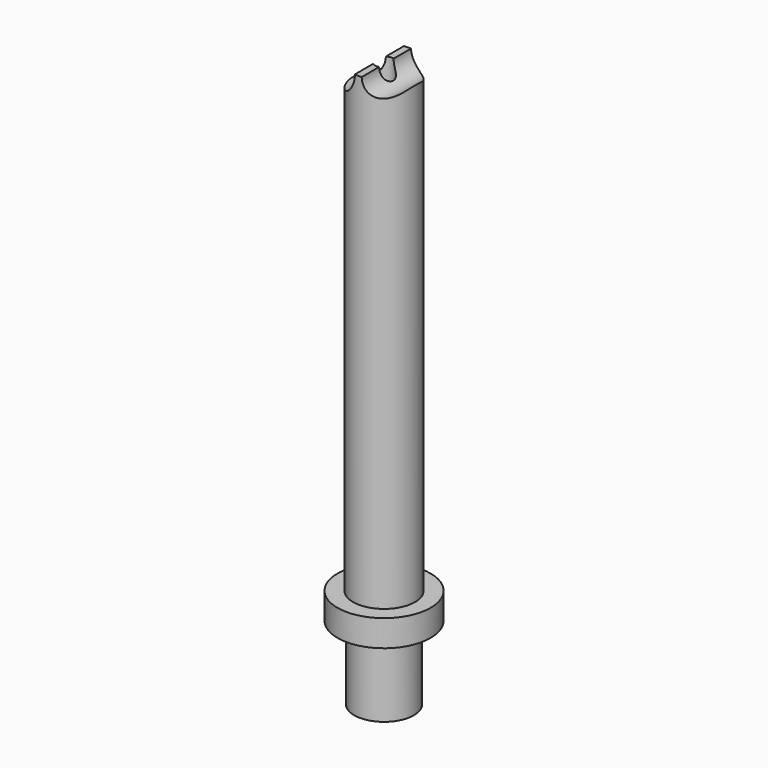
from build123d import *

# Parameters (mm, degrees)
F0_R      = 3.325
F1_DEPTH  = 50
F2_R      = 5
F2_R_2    = 3.325
F3_DEPTH  = 2.85
F4_R      = 3.2
F5_DEPTH  = 7.9
F6_R      = 1
F7_DEPTH  = 55
F8_R      = 2.05
F9_DEPTH  = 6.9
F10_R     = 2.5
F10_R_2   = 1.75
F11_DEPTH = 4


with BuildPart() as f1:
    # F0 (on Top) → F1 (new body)
    with BuildSketch(Plane.XY):
        Circle(F0_R)
    extrude(amount=F1_DEPTH)

    # F2 (on face) → F3 (join)
    with BuildSketch(Plane.XY):
        Circle(F2_R)
        Circle(F2_R_2, mode=Mode.SUBTRACT)
        Circle(F2_R)
    extrude(amount=-F3_DEPTH)

    # F4 (on face) → F5 (join)
    with BuildSketch(Plane(origin=(0, 0, -2.85), x_dir=(1, 0, 0), z_dir=(0, 0, -1))):
        Circle(F4_R)
    extrude(amount=F5_DEPTH)

    # F6 (on face) → F7 (cut)
    with BuildSketch(Plane.XY.offset(50)):
        Circle(F6_R)
    extrude(amount=-F7_DEPTH, mode=Mode.SUBTRACT)

    # F8 (on face) → F9 (cut)
    with BuildSketch(Plane(origin=(0, 0, -10.75), x_dir=(1, 0, 0), z_dir=(0, 0, -1))):
        Circle(F8_R)
    extrude(amount=-F9_DEPTH, mode=Mode.SUBTRACT)

    # F10 (on Front) → F11 (cut, symmetric)
    with BuildSketch(Plane.XZ):
        with Locations((-3, 50)):
            Circle(F10_R)
        with Locations((2, 50)):
            Circle(F10_R_2)
    extrude(amount=F11_DEPTH, both=True, mode=Mode.SUBTRACT)


solid = f1.part
